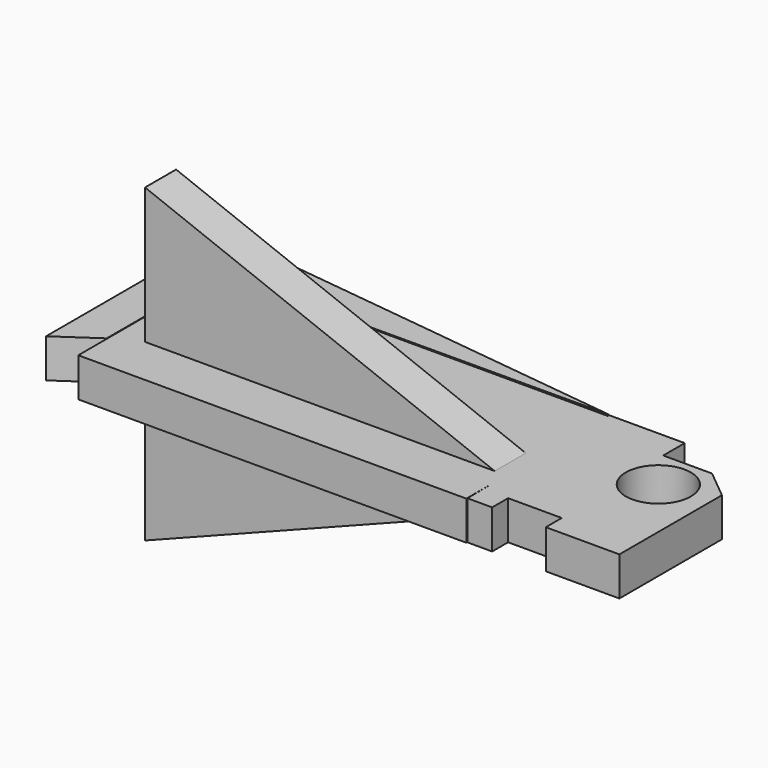
from build123d import *

# Parameters (mm, degrees)
F0_W     = 253.6633908749
F0_H     = 116.4356470108
F5_DEPTH = 25.4
F8_DEPTH = 25.4
F1_R     = 21.2689966395
F9_DEPTH = 25.4


# Not quite as in the source:
# - a feature of the source that left no trace in its solid (it failed there, or was rolled back) is left out


with BuildPart() as f5:
    # F0 (on Top) → F5 (new body)
    with BuildSketch(Plane.XY):
        Rectangle(F0_W, F0_H)
    extrude(amount=F5_DEPTH)

    # F7 (on Front) → F8 (join)
    with BuildSketch(Plane.XZ):
        Polygon((-109.4650974564, 25.4), (-109.4650974564, 0), (-109.4650974564, -88.9), (119.1349025436, 0), (119.1349025436, 25.4), (-109.4650974564, 114.3), align=None)
    extrude(amount=F8_DEPTH)

    # F1 (on Top) → F9 (join)
    with BuildSketch(Plane.XY):
        Polygon((175.5617409945, 59.3426562846), (126.1054128408, 59.3426562846), (127.0046085119, -57.5541220605), (143.1903243065, -57.5541220605), (143.1903243065, -44.5156358182), (178.25935781, -44.5156358182), (178.25935781, -57.5541220605), (226.3668775558, -57.5541220605), (226.3668775558, -44.5156358182), (226.3668775558, -17.5394564867), (226.3668775558, 0), (226.3668775558, 26.2293902971), (207.4835598469, 41.8081395328), (175.5617409945, 41.8081395328), align=None)
        with Locations((193.577849129, 15.2662187056)):
            Circle(F1_R, mode=Mode.SUBTRACT)
    extrude(amount=F9_DEPTH)


with BuildPart() as f5b:
    # F3 (on Top) → F5, piece 2 (new body)
    with BuildSketch(Plane.XY):
        Polygon((-127.4706870317, 90.36526829), (-127.4706870317, 58.8930547237), (125.6558001041, 59.7922615707), align=None)
    extrude(amount=F5_DEPTH)


with BuildPart() as f5c:
    # F4 (on Top) → F5, piece 3 (new body)
    with BuildSketch(Plane.XY):
        Polygon((-152.8075635433, -52.0751588047), (-127.2091120481, -34.560430795), (-127.2091120481, 32.8039005399), (-152.8075635433, 57.7287077904), align=None)
    extrude(amount=F5_DEPTH)


solid = Compound([f5.part, f5b.part, f5c.part])
